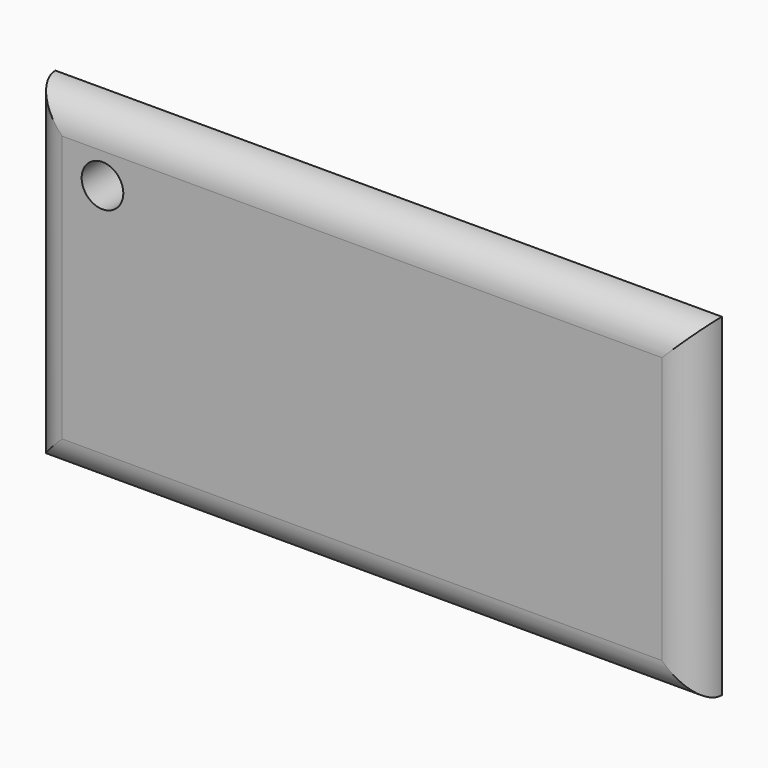
from build123d import *

# Parameters (mm, degrees)
F1_DEPTH    = 3.175
F2_R        = 5.08
F3_R        = 3.175
F4_DEPTH    = 25.4
F5_T1_DEPTH = 118.410793948
F5_T3_DEPTH = 67.600521864
F5_T5_DEPTH = 118.4005208253
F5_T7_DEPTH = 67.6005208253


# Not quite as in the source:
# - a fillet or chamfer that OpenCascade refuses, or shapes differently, is made with other operations: its cross-section is extruded or revolved along the edge and cut away or added


with BuildPart() as f1:
    # F0 (on Front) → F1 (new body, symmetric)
    with BuildSketch(Plane.XZ):
        Polygon((52.0995333791, 24.9929322481), (-49.5107397437, 24.9929322481), (-49.5107397437, -25.8070677519), (52.0892602563, -25.8070677519), align=None)
    extrude(amount=F1_DEPTH, both=True)

    # F2
    f2_edges = [f1.edges().sort_by_distance(p)[0] for p in [
        (-49.51074, -3.175, -0.407068),
        (1.294397, -3.175, 24.992932),
        (52.094397, -3.175, -0.407068),
        (1.28926, -3.175, -25.807068),
    ]]
    fillet(f2_edges, radius=F2_R)

    # F3 (on face) → F4 (cut)
    with BuildSketch(Plane.XZ.offset(3.175)):
        with Locations((-38.2700785995, 15.264518559)):
            Circle(F3_R)
    extrude(amount=-F4_DEPTH, mode=Mode.SUBTRACT)

    # F5: fillet of radius 5.08 on 4 edges, made by hand

    # F5_s2 → F5_t1 (cut)
    with BuildSketch(Plane.YZ.offset(-57.9110001563)):
        with BuildLine():
            ThreePointArc((1.905, 24.9929322481), (2.8469048812, 23.4288793073), (3.175, 21.6328280831))
            Line((3.175, 21.6328280831), (3.175, 24.9929322481))
            Line((3.175, 24.9929322481), (1.905, 24.9929322481))
        make_face()
    extrude(amount=F5_T1_DEPTH, mode=Mode.SUBTRACT)

    # F5_s4 → F5_t3 (cut)
    with BuildSketch(Plane(origin=(-0.0069155089, 0, -34.196793092), x_dir=(0, 1, 0), z_dir=(0.0002022268, 0, 0.9999999796))):
        with BuildLine():
            ThreePointArc((3.175, -48.7343739074), (2.8469048812, -50.5304251316), (1.905, -52.0944780725))
            Line((1.905, -52.0944780725), (3.175, -52.0944780725))
            Line((3.175, -52.0944780725), (3.175, -48.7343739074))
        make_face()
    extrude(amount=F5_T3_DEPTH, mode=Mode.SUBTRACT)

    # F5_s6 → F5_t5 (cut)
    with BuildSketch(Plane.YZ.offset(-57.9110001563)):
        with BuildLine():
            ThreePointArc((3.175, -22.4469635868), (2.8469048812, -24.243014811), (1.905, -25.8070677519))
            Line((1.905, -25.8070677519), (3.175, -25.8070677519))
            Line((3.175, -25.8070677519), (3.175, -22.4469635868))
        make_face()
    extrude(amount=F5_T5_DEPTH, mode=Mode.SUBTRACT)

    # F5_s8 → F5_t7 (cut)
    with BuildSketch(Plane.XY.offset(-34.2073281645)):
        with BuildLine():
            ThreePointArc((-49.5107397437, 1.905), (-47.9466868029, 2.8469048812), (-46.1506355787, 3.175))
            Line((-46.1506355787, 3.175), (-49.5107397437, 3.175))
            Line((-49.5107397437, 3.175), (-49.5107397437, 1.905))
        make_face()
    extrude(amount=F5_T7_DEPTH, mode=Mode.SUBTRACT)


solid = f1.part
